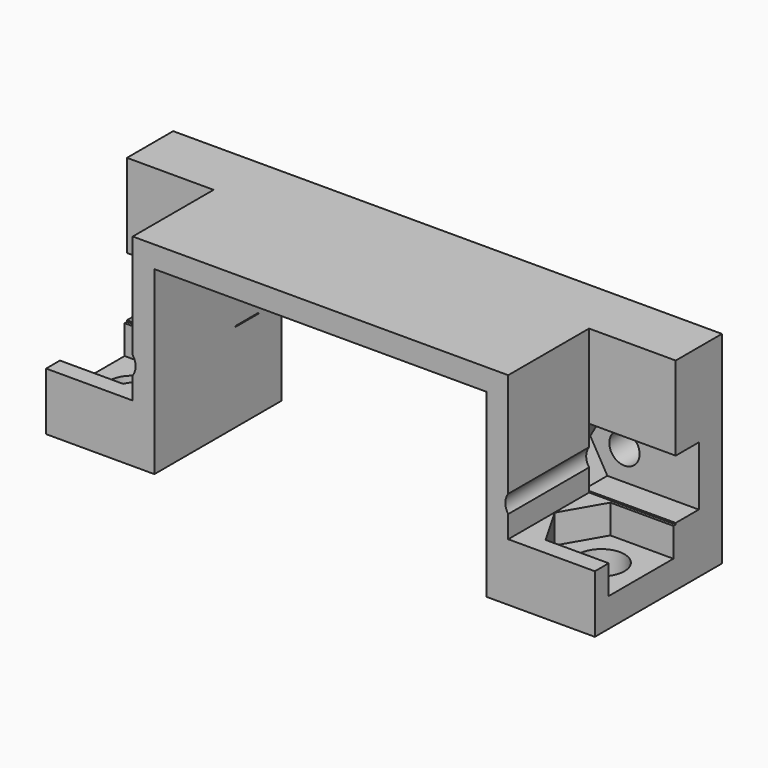
from build123d import *

# Parameters (mm, degrees)
F1_DEPTH        = 11
F2_W            = 6
F2_H            = 10
F3_DEPTH        = 4
F4_R            = 1.05
F5_DEPTH        = 11
F5_COPIES_COUNT = 2
F5_COPIES_PITCH = 27.7
F7_DEPTH        = 2
F8_R            = 1.6
F9_DEPTH        = 4
F11_DEPTH       = 2


# Not quite as in the source:
# - a pattern or mirror of a feature is missing from the dataset's text; its kind, count and spacing are read off the source's solid


with BuildPart() as f1:
    # F0 (on Front) → F1 (new body)
    with BuildSketch(Plane.XZ):
        Polygon((-19, 4), (-19, 0), (-11.5, 0), (-11.5, 12.5), (11.5, 12.5), (11.5, 0), (19, 0), (19, 4), (13, 4), (13, 14), (-13, 14), (-13, 4), align=None)
    extrude(amount=F1_DEPTH)

    # F2 (on face) → F3 (join)
    with BuildSketch(Plane(origin=(0, 0, 0), x_dir=(-1, 0, 0), z_dir=(0, 1, 0))):
        with Locations((-16, 9)):
            Rectangle(F2_W, F2_H)
        with Locations((16, 9)):
            Rectangle(F2_W, F2_H)
    extrude(amount=-F3_DEPTH)

    # F4 (on Front) → F5 (cut, through all)
    with BuildSketch(Plane.XZ):
        with Locations((-13.85, 6.15)):
            Circle(F4_R)
    f5 = extrude(amount=F5_DEPTH, mode=Mode.SUBTRACT)

    # F5_copies: F5 ×2
    with Locations(*[(i * F5_COPIES_PITCH, 0, 0) for i in range(1, F5_COPIES_COUNT)]):
        add(f5, mode=Mode.SUBTRACT)

    # F6 (on face) → F7 (cut)
    with BuildSketch(Plane.XZ.offset(4)):
        Polygon((-12.6664319482, 8.2), (-15.0335680518, 8.2), (-16.2171361037, 6.15), (-15.0335680518, 4.1), (-12.6664319482, 4.1), (-11.4828638963, 6.15), align=None)
        Polygon((-16.2171361037, 6.15), (-15.0335680518, 8.2), (-19, 8.2), (-19, 4.1), (-15.0335680518, 4.1), align=None)
    f7 = extrude(amount=-F7_DEPTH, mode=Mode.SUBTRACT)

    # F7_copies: F7 across plane
    add(f7.mirror(Plane(origin=(0, 0, 0), x_dir=(0, 0, 1), z_dir=(1, 0, 0))), mode=Mode.SUBTRACT)

    # F8 (on face) → F9 (cut, through all)
    with BuildSketch(Plane(origin=(0, 0, 0), x_dir=(1, 0, 0), z_dir=(0, 0, -1))):
        with Locations((-16.25, 7)):
            Circle(F8_R)
    f9 = extrude(amount=-F9_DEPTH, mode=Mode.SUBTRACT)

    # F9_copies: F9 across plane
    add(f9.mirror(Plane(origin=(0, 0, 0), x_dir=(0, 0, 1), z_dir=(1, 0, 0))), mode=Mode.SUBTRACT)

    # F10 (on face) → F11 (cut)
    with BuildSketch(Plane.XY.offset(4)):
        Polygon((-14.6334192463, -4.2), (-17.8665807537, -4.2), (-19, -6.1631397208), (-19, -7.8368602792), (-17.8665807537, -9.8), (-14.6334192463, -9.8), (-13.0168384925, -7), align=None)
        Polygon((-19, -6.1631397208), (-17.8665807537, -4.2), (-19, -4.2), align=None)
        Polygon((-19, -7.8368602792), (-19, -6.1631397208), (-19.4831615075, -7), align=None)
        Polygon((-17.8665807537, -9.8), (-19, -7.8368602792), (-19, -9.8), align=None)
    f11 = extrude(amount=-F11_DEPTH, mode=Mode.SUBTRACT)

    # F11_copies: F11 across plane
    add(f11.mirror(Plane(origin=(0, 0, 0), x_dir=(0, 0, 1), z_dir=(1, 0, 0))), mode=Mode.SUBTRACT)


solid = f1.part
